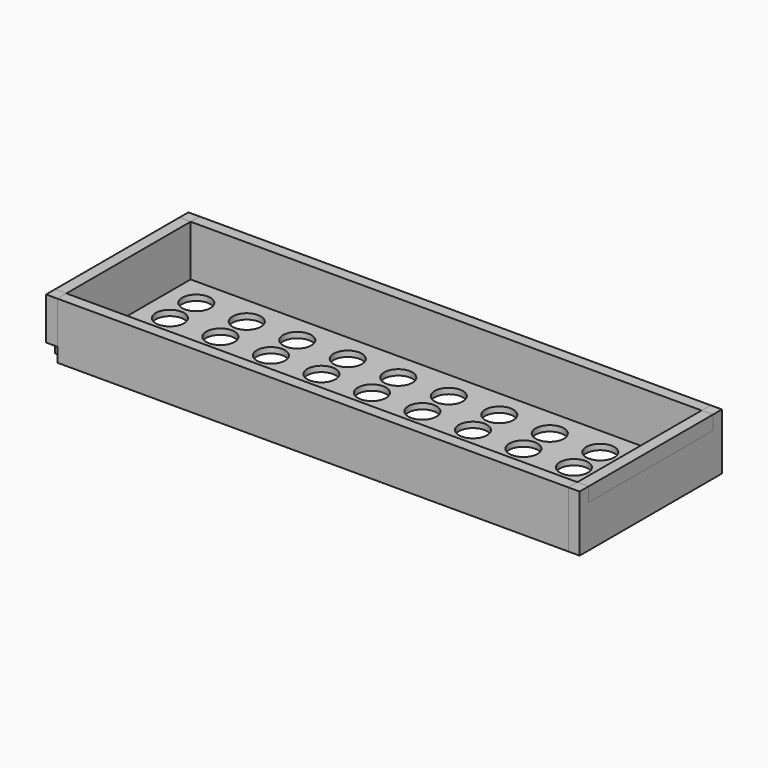
from build123d import *

# Parameters (mm, degrees)
F0_W     = 4
F0_H     = 55
F1_DEPTH = 20
F0_W_2   = 181
F0_H_2   = 4
F2_START = 5
F2_DEPTH = 15
F0_R     = 5
F3_DEPTH = 2
F4_DEPTH = 15
F5_DEPTH = 20


with BuildPart() as f1:
    # F0 (on Top) → F1 (new body)
    with BuildSketch(Plane.XY):
        with Locations((-86.6956989169, 0)):
            Rectangle(F0_W, F0_H)
    extrude(amount=F1_DEPTH)


with BuildPart() as f1b:
    # F0 (on Top) → F1, piece 2 (new body)
    with BuildSketch(Plane.XY):
        with Locations((5.8043010831, -29.5)):
            Rectangle(F0_W_2, F0_H_2)
    extrude(amount=F1_DEPTH)


with BuildPart() as f1c:
    # F0 (on Top) → F1, piece 3 (new body)
    with BuildSketch(Plane.XY):
        with Locations((5.8043010831, 29.5)):
            Rectangle(F0_W_2, F0_H_2)
    extrude(amount=F1_DEPTH)


with BuildPart() as f1d:
    # F0 (on Top) → F1, piece 4 (new body)
    with BuildSketch(Plane.XY):
        with Locations((98.3043010831, 0)):
            Rectangle(F0_W, F0_H)
    extrude(amount=F1_DEPTH)


with BuildPart() as f2:
    # F0 (on Top) → F2 (new body)
    with BuildSketch(Plane.XY.offset(F2_START)):
        with Locations((98.3043010831, 29.5)):
            Rectangle(F0_W, F0_H_2)
    extrude(amount=F2_DEPTH)


with BuildPart() as f2b:
    # F0 (on Top) → F2, piece 2 (new body)
    with BuildSketch(Plane.XY.offset(F2_START)):
        with Locations((98.3043010831, -29.5)):
            Rectangle(F0_W, F0_H_2)
    extrude(amount=F2_DEPTH)


with BuildPart() as f2c:
    # F0 (on Top) → F2, piece 3 (new body)
    with BuildSketch(Plane.XY.offset(F2_START)):
        with Locations((-86.6956989169, -29.5)):
            Rectangle(F0_W, F0_H_2)
    extrude(amount=F2_DEPTH)


with BuildPart() as f2d:
    # F0 (on Top) → F2, piece 4 (new body)
    with BuildSketch(Plane.XY.offset(F2_START)):
        with Locations((-86.6956989169, 29.5)):
            Rectangle(F0_W, F0_H_2)
    extrude(amount=F2_DEPTH)


with BuildPart() as f3:
    # F0 (on Top) → F3 (new body)
    with BuildSketch(Plane.XY):
        with Locations((5.8043010831, 0)):
            Rectangle(F0_W_2, F0_H)
        with Locations((-74.6956989169, -17.5)):
            Circle(F0_R, mode=Mode.SUBTRACT)
        with Locations((-56.806810028, -17.5)):
            Circle(F0_R, mode=Mode.SUBTRACT)
        with Locations((-38.9179211391, -17.5)):
            Circle(F0_R, mode=Mode.SUBTRACT)
        with Locations((-21.0290322502, -17.5)):
            Circle(F0_R, mode=Mode.SUBTRACT)
        with Locations((-3.1401433614, -17.5)):
            Circle(F0_R, mode=Mode.SUBTRACT)
        with Locations((-74.6956989169, -5.8333333333)):
            Circle(F0_R, mode=Mode.SUBTRACT)
        with Locations((-56.806810028, -5.8333333333)):
            Circle(F0_R, mode=Mode.SUBTRACT)
        with Locations((-38.9179211391, -5.8333333333)):
            Circle(F0_R, mode=Mode.SUBTRACT)
        with Locations((-21.0290322502, -5.8333333333)):
            Circle(F0_R, mode=Mode.SUBTRACT)
        with Locations((-3.1401433614, -5.8333333333)):
            Circle(F0_R, mode=Mode.SUBTRACT)
        with Locations((14.7487455275, -17.5)):
            Circle(F0_R, mode=Mode.SUBTRACT)
        with Locations((32.6376344164, -17.5)):
            Circle(F0_R, mode=Mode.SUBTRACT)
        with Locations((50.5265233053, -17.5)):
            Circle(F0_R, mode=Mode.SUBTRACT)
        with Locations((68.4154121942, -17.5)):
            Circle(F0_R, mode=Mode.SUBTRACT)
        with Locations((86.3043010831, -17.5)):
            Circle(F0_R, mode=Mode.SUBTRACT)
        with Locations((14.7487455275, -5.8333333333)):
            Circle(F0_R, mode=Mode.SUBTRACT)
        with Locations((32.6376344164, -5.8333333333)):
            Circle(F0_R, mode=Mode.SUBTRACT)
        with Locations((50.5265233053, -5.8333333333)):
            Circle(F0_R, mode=Mode.SUBTRACT)
        with Locations((68.4154121942, -5.8333333333)):
            Circle(F0_R, mode=Mode.SUBTRACT)
        with Locations((86.3043010831, -5.8333333333)):
            Circle(F0_R, mode=Mode.SUBTRACT)
        with Locations((-74.6956989169, 5.8333333333)):
            Circle(F0_R, mode=Mode.SUBTRACT)
        with Locations((-56.806810028, 5.8333333333)):
            Circle(F0_R, mode=Mode.SUBTRACT)
        with Locations((-38.9179211391, 5.8333333333)):
            Circle(F0_R, mode=Mode.SUBTRACT)
        with Locations((-21.0290322502, 5.8333333333)):
            Circle(F0_R, mode=Mode.SUBTRACT)
        with Locations((-3.1401433614, 5.8333333333)):
            Circle(F0_R, mode=Mode.SUBTRACT)
        with Locations((-74.6956989169, 17.5)):
            Circle(F0_R, mode=Mode.SUBTRACT)
        with Locations((-56.806810028, 17.5)):
            Circle(F0_R, mode=Mode.SUBTRACT)
        with Locations((-38.9179211391, 17.5)):
            Circle(F0_R, mode=Mode.SUBTRACT)
        with Locations((-21.0290322502, 17.5)):
            Circle(F0_R, mode=Mode.SUBTRACT)
        with Locations((-3.1401433614, 17.5)):
            Circle(F0_R, mode=Mode.SUBTRACT)
        with Locations((14.7487455275, 5.8333333333)):
            Circle(F0_R, mode=Mode.SUBTRACT)
        with Locations((32.6376344164, 5.8333333333)):
            Circle(F0_R, mode=Mode.SUBTRACT)
        with Locations((50.5265233053, 5.8333333333)):
            Circle(F0_R, mode=Mode.SUBTRACT)
        with Locations((68.4154121942, 5.8333333333)):
            Circle(F0_R, mode=Mode.SUBTRACT)
        with Locations((86.3043010831, 5.8333333333)):
            Circle(F0_R, mode=Mode.SUBTRACT)
        with Locations((14.7487455275, 17.5)):
            Circle(F0_R, mode=Mode.SUBTRACT)
        with Locations((32.6376344164, 17.5)):
            Circle(F0_R, mode=Mode.SUBTRACT)
        with Locations((50.5265233053, 17.5)):
            Circle(F0_R, mode=Mode.SUBTRACT)
        with Locations((68.4154121942, 17.5)):
            Circle(F0_R, mode=Mode.SUBTRACT)
        with Locations((86.3043010831, 17.5)):
            Circle(F0_R, mode=Mode.SUBTRACT)
    extrude(amount=F3_DEPTH)


with BuildPart() as f4:
    # F0 (on Top) → F4 (new body)
    with BuildSketch(Plane.XY):
        with Locations((98.3043010831, 0)):
            Rectangle(F0_W, F0_H)
    extrude(amount=F4_DEPTH)

    # F0 (on Top) → F5 (join)
    with BuildSketch(Plane.XY):
        with Locations((98.3043010831, 29.5)):
            Rectangle(F0_W, F0_H_2)
        with Locations((98.3043010831, -29.5)):
            Rectangle(F0_W, F0_H_2)
    extrude(amount=F5_DEPTH)


solid = Compound([f1.part, f1b.part, f1c.part, f1d.part, f2.part, f2b.part, f2c.part, f2d.part, f3.part, f4.part])
